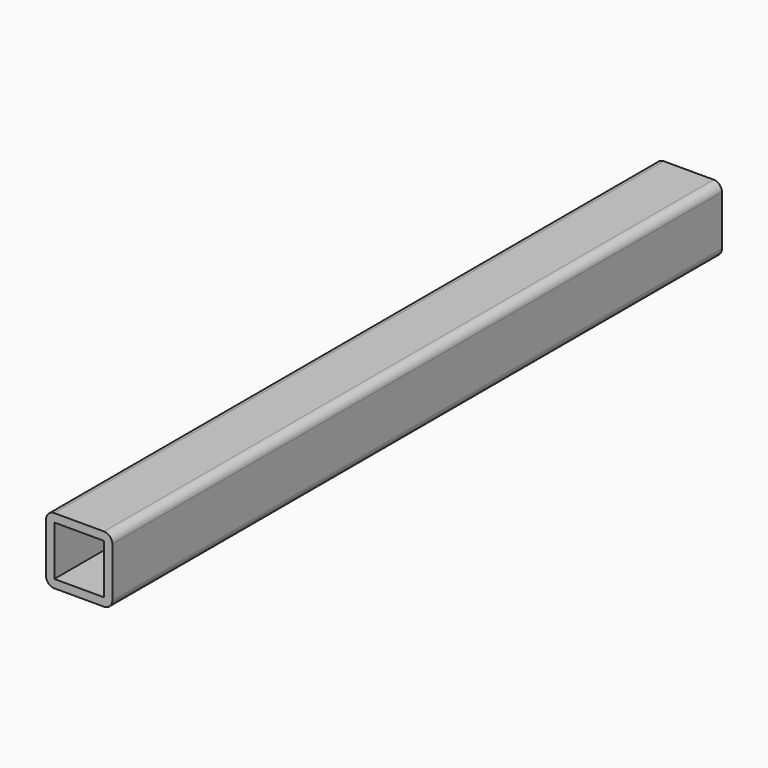
from build123d import *

# Parameters (mm, degrees)
F0_W     = 25.4
F0_H     = 25.4
F1_DEPTH = 292.1
F2_R     = 3.175
F3_T     = 3.175


# Not quite as in the source:
# - a shell that OpenCascade refuses in one call is made with other operations: the cavity is built on its own and cut out


with BuildPart() as f1:
    # F0 (on Front) → F1 (new body)
    with BuildSketch(Plane.XZ):
        Rectangle(F0_W, F0_H)
    extrude(amount=F1_DEPTH)

    # F2
    f2_edges = [f1.edges().sort_by_distance(p)[0] for p in [
        (-12.7, -146.05, 12.7),
        (12.7, -146.05, 12.7),
        (12.7, -146.05, -12.7),
        (-12.7, -146.05, -12.7),
    ]]
    fillet(f2_edges, radius=F2_R)

    # F3: shell of thickness 3.175, made by hand


with BuildPart() as f3_core1:
    # F3_t2: copy of F1
    add(f1.part)

    # the walls: a layer under each face that stays
    f3_faces = [f3_core1.faces().sort_by_distance(p)[0] for p in [
        (0, -146.05, -12.7),
        (-12.7, -146.05, 0),
        (12.7, -146.05, 0),
        (0, -146.05, 12.7),
    ]]
    thicken(f3_faces, amount=-F3_T, mode=Mode.SUBTRACT)


with BuildPart() as f1_1:
    add(f1.part)

    # what is left inside the walls is the cavity
    f3_cavity = [f3_core1.part.solids().sort_by_distance(p)[0] for p in [
        (0, -194.733333, -9.49325),
    ]]
    add(f3_cavity, mode=Mode.SUBTRACT)


solid = f1_1.part
